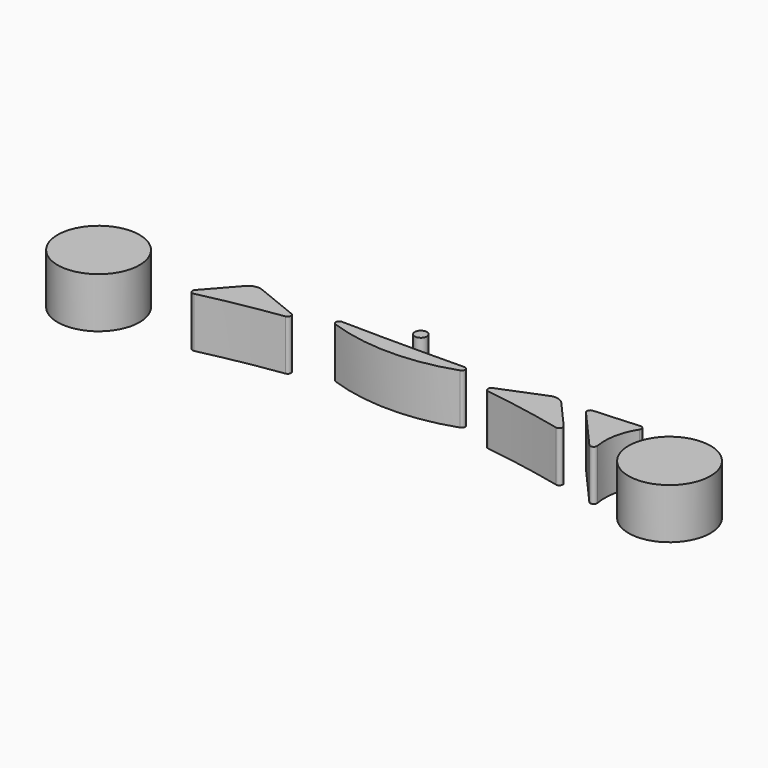
from build123d import *

# Parameters (mm, degrees)
F0_R     = 20.6756
F1_DEPTH = 25.4
F0_R_2   = 3.0734


# Not quite as in the source:
# - ends of sketch curves that miss each other by under 0.0002 mm in the source are joined
# - a feature of the source that left no trace in its solid (it failed there, or was rolled back) is left out


with BuildPart() as f1:
    # F0 (on Top) → F1 (new body)
    with BuildSketch(Plane.XY):
        Circle(F0_R)
    extrude(amount=F1_DEPTH)


with BuildPart() as f1b:
    # F0 (on Top) → F1, piece 2 (new body)
    with BuildSketch(Plane.XY):
        with Locations((288.0868, 0)):
            Circle(F0_R)
    extrude(amount=F1_DEPTH)


with BuildPart() as f1c:
    # F0 (on Top) → F1, piece 3 (new body)
    with BuildSketch(Plane.XY):
        with BuildLine():
            Line((64.3141716, 12.1225818), (51.0722372, -2.9026612))
            ThreePointArc((51.0722372, -2.9026612), (50.886637197, -4.8983229131), (52.7293898046, -5.6865968893))
            ThreePointArc((52.7293898046, -5.6865968893), (72.7281380064, -1.5489138472), (92.885832563, 1.728361878))
            ThreePointArc((92.885832563, 1.728361878), (94.3380072647, 3.2062647833), (93.2864207732, 4.9914536905))
            Line((93.2864207732, 4.9914536905), (71.4569801787, 13.8116269873))
            ThreePointArc((71.4569801787, 13.8116269873), (67.6168206872, 14.1036419642), (64.3141716, 12.1225818))
        make_face()
    extrude(amount=F1_DEPTH)


with BuildPart() as f1d:
    # F0 (on Top) → F1, piece 4 (new body)
    with BuildSketch(Plane.XY):
        with BuildLine():
            ThreePointArc((235.3574089318, -5.6866037007), (237.2001615394, -4.8983297245), (237.0145615364, -2.9026680114))
            Line((237.0145615364, -2.9026680114), (223.7726271364, 12.1225749886))
            ThreePointArc((223.7726271364, 12.1225749886), (220.4699709207, 14.1036432413), (216.6298123513, 13.8116286368))
            Line((216.6298123513, 13.8116286368), (194.8003724, 4.9914556))
            ThreePointArc((194.8003724, 4.9914556), (193.7487857413, 3.2062666252), (195.2008776796, 1.7283753619))
            ThreePointArc((195.2008776796, 1.7283753619), (215.3585722363, -1.5489003634), (235.3574089318, -5.6866037007))
        make_face()
    extrude(amount=F1_DEPTH)


with BuildPart() as f1e:
    # F0 (on Top) → F1, piece 5 (new body)
    with BuildSketch(Plane.XY):
        with BuildLine():
            ThreePointArc((260.5652400713, 16.0522893388), (249.1287669286, 15.2867037282), (237.6874855708, 14.596689118))
            ThreePointArc((237.6874855708, 14.596689118), (236.2140385559, 13.5536732496), (236.5075745699, 11.7724475997))
            Line((236.5075745699, 11.7724475997), (254.9323832, -9.1336622))
            ThreePointArc((254.9323832, -9.1336622), (256.947957492, -9.5415132252), (257.8846881323, -7.7108254055))
            ThreePointArc((257.8846881323, -7.7108254055), (258.0038440306, 3.2617628688), (262.1165200814, 13.4351540637))
            ThreePointArc((262.1165200814, 13.4351540637), (262.1484797054, 15.2224111463), (260.5652400713, 16.0522893388))
        make_face()
    extrude(amount=F1_DEPTH)


with BuildPart() as f1f:
    # F0 (on Top) → F1, piece 6 (new body)
    with BuildSketch(Plane.XY):
        with BuildLine():
            ThreePointArc((174.8717102393, 12.0594991546), (144.0434, 11.7855877651), (113.2150897607, 12.0594991546))
            ThreePointArc((113.2150897607, 12.0594991546), (111.5097977558, 10.6584288913), (112.6218159145, 8.7520098426))
            ThreePointArc((112.6218159145, 8.7520098426), (144.0434, 3.403589621), (175.4649807504, 8.7520086732))
            ThreePointArc((175.4649807504, 8.7520086732), (176.5770022442, 10.6584288913), (174.8717102393, 12.0594991546))
        make_face()
    extrude(amount=F1_DEPTH)


with BuildPart() as f1g:
    # F0 (on Top) → F1, piece 7 (new body)
    with BuildSketch(Plane.XY):
        with Locations((144.0434, 23.1902)):
            Circle(F0_R_2)
    extrude(amount=F1_DEPTH)


solid = Compound([f1.part, f1b.part, f1c.part, f1d.part, f1e.part, f1f.part, f1g.part])
